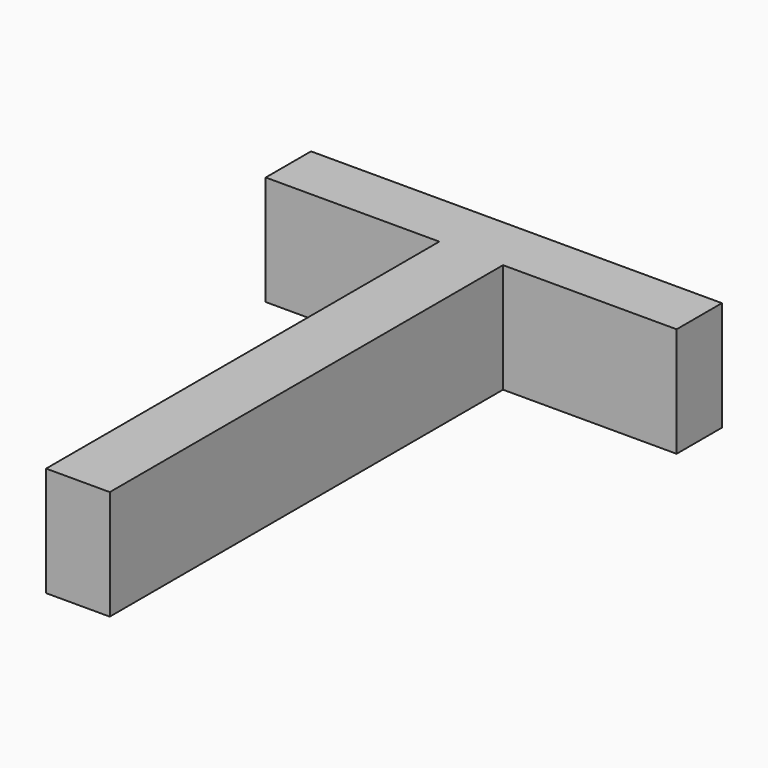
from build123d import *

# Parameters (mm, degrees)
F0_TEXT_SIZE = 177.868284906
F1_DEPTH     = 25.4


# Not quite as in the source:
# - Text() gives the source's letters only with a copy of the font that has no kerning and outlines rounded to 1/6400 em; it was checked with that copy


with BuildPart() as f1:
    # F0 (on Top) → F1 (new body)
    with BuildSketch(Plane.XY):
        with Locations((-59.6080645919, -60.4683868587)):
            Text('T', F0_TEXT_SIZE, font='Open Sans', text_align=(TextAlign.LEFT, TextAlign.BOTTOM))
    extrude(amount=F1_DEPTH)


solid = f1.part
